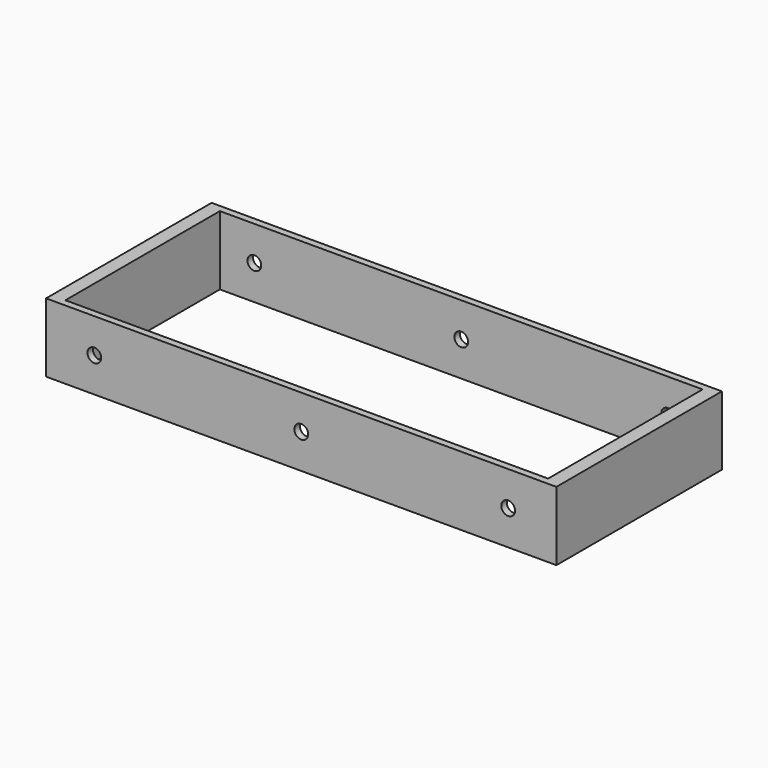
from build123d import *

# Parameters (mm, degrees)
F0_W     = 1879.6
F0_H     = 762
F1_DEPTH = 127
F2_W     = 1778
F2_H     = 711.2
F3_DEPTH = 635
F4_R     = 25.4
F5_DEPTH = 762.001


# Not quite as in the source:
# - a feature names something its author has since deleted; it is built from what else it names


with BuildPart() as f1:
    # F0 (on Top) → F1 (new body, symmetric)
    with BuildSketch(Plane.XY):
        Rectangle(F0_W, F0_H)
    extrude(amount=F1_DEPTH, both=True)

    # F2 (on face) → F3 (cut, symmetric)
    with BuildSketch(Plane.XY.offset(127)):
        Rectangle(F2_W, F2_H)
    extrude(amount=F3_DEPTH, both=True, mode=Mode.SUBTRACT)

    # F4 (on face) → F5 (cut, through all)
    with BuildSketch(Plane.XZ.offset(381)):
        with Locations((-762, 0)):
            Circle(F4_R)
        with Locations((762, 0)):
            Circle(F4_R)
        Circle(F4_R)
    extrude(amount=-F5_DEPTH, mode=Mode.SUBTRACT)


solid = f1.part
